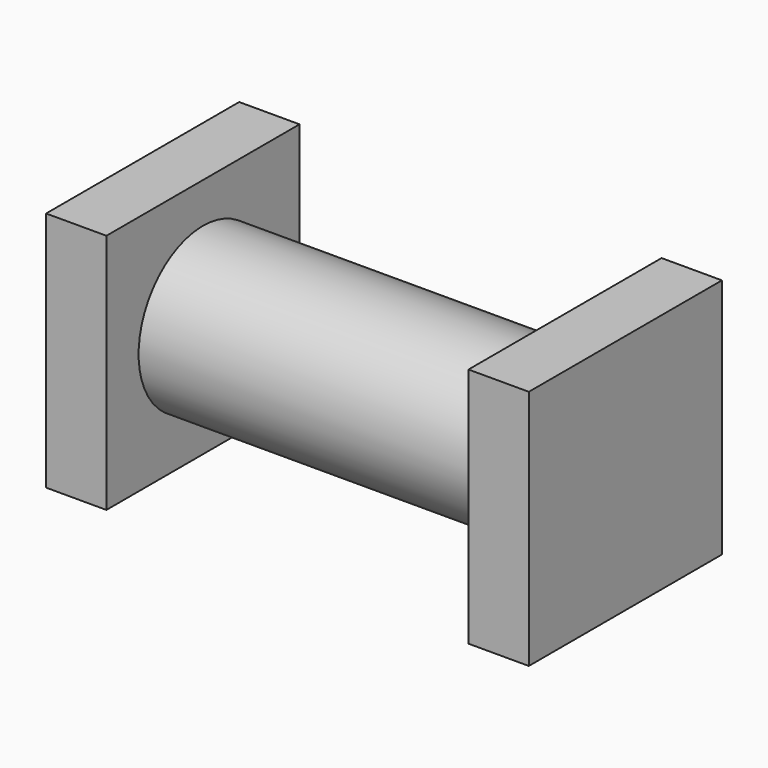
from build123d import *

# Parameters (mm, degrees)
F0_W     = 76.2
F0_H     = 76.2
F1_DEPTH = 19.05
F4_R     = 25.4
F5_DEPTH = 152.4


# Not quite as in the source:
# - a feature names something its author has since deleted; it is built from what else it names


with BuildPart() as f1:
    # F0 (on Right) → F1 (new body)
    with BuildSketch(Plane.YZ):
        Rectangle(F0_W, F0_H)
    extrude(amount=F1_DEPTH)


with BuildPart() as f1_1:
    # F2: moved
    add(f1.part.moved(Location((-76.2, 0, 0))))


with BuildPart() as f3_1:
    # F3: instance of F1
    add(f1_1.part.mirror(Plane.YZ))

    # F4 (on face) → F5 (join)
    with BuildSketch(Plane.YZ.offset(76.2)):
        Circle(F4_R)
    extrude(amount=-F5_DEPTH)


solid = Compound([f1_1.part, f3_1.part])
